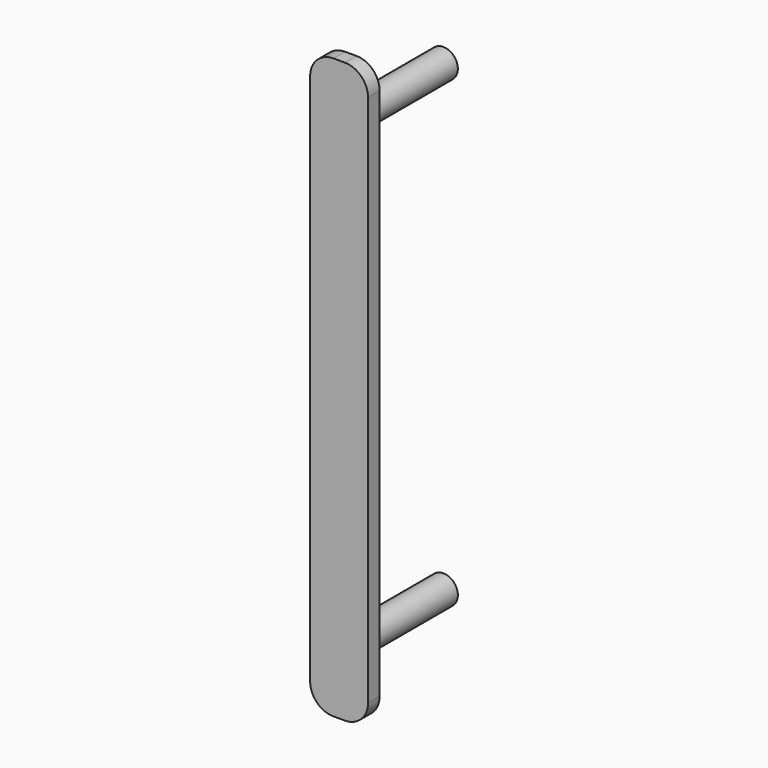
from build123d import *

# Parameters (mm, degrees)
F0_R     = 3.175
F1_DEPTH = 25.4
F3_DEPTH = 3.175
F4_R     = 5.08


with BuildPart() as f1:
    # F0 (on Front) → F1 (new body)
    with BuildSketch(Plane.XZ):
        with Locations((0, 101.6)):
            Circle(F0_R)
    extrude(amount=F1_DEPTH)


with BuildPart() as f1b:
    # F0 (on Front) → F1, piece 2 (new body)
    with BuildSketch(Plane.XZ):
        Circle(F0_R)
    extrude(amount=F1_DEPTH)

    # F2 (on face) → F3 (join)
    with BuildSketch(Plane.XZ.offset(25.4)):
        Polygon((-6.35, -13.2284704596), (0, -13.2284704596), (6.35, -13.2284704596), (6.35, 113.7715295404), (0, 113.7715295404), (-6.35, 113.7715295404), align=None)
    extrude(amount=F3_DEPTH)

    # F4
    f4_edges = [f1b.edges().sort_by_distance(p)[0] for p in [
        (-6.35, -26.9875, 113.77153),
        (6.35, -26.9875, 113.77153),
        (6.35, -26.9875, -13.22847),
        (-6.35, -26.9875, -13.22847),
    ]]
    fillet(f4_edges, radius=F4_R)


solid = Compound([f1.part, f1b.part])
